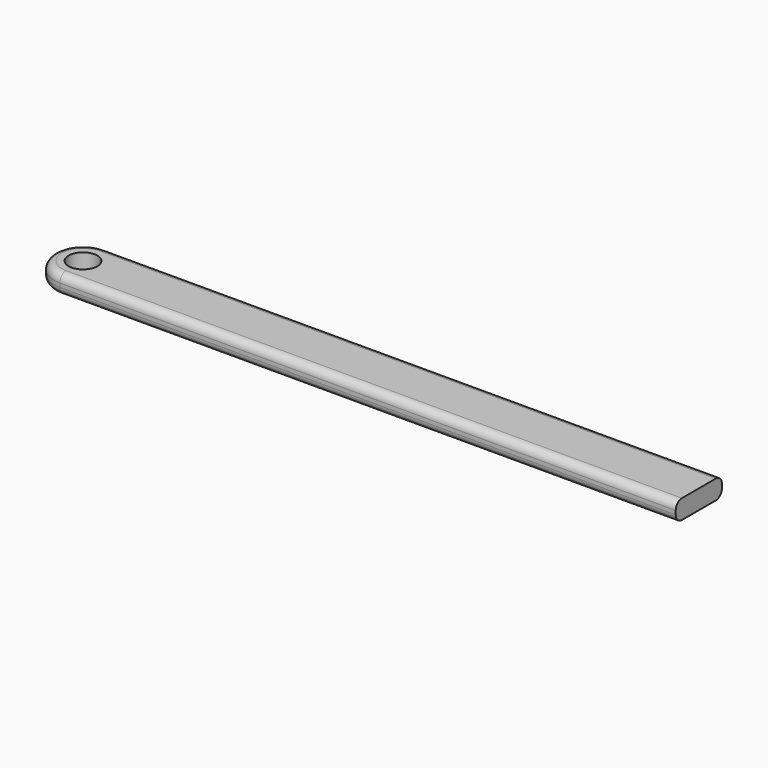
from build123d import *

# Parameters (mm, degrees)
F0_R     = 4.7625
F2_DEPTH = 3.175
F3_R     = 2.54


# Not quite as in the source:
# - a variable given as a bare number and used for a length is read in inches; the dataset says mm whatever the document's units were


with BuildPart() as f2:
    # F0 (on Top) → F2 (new body, symmetric)
    with BuildSketch(Plane.XY):
        with BuildLine():
            Line((-203.2, 0), (0, 0))
            Line((0, 0), (0, 19.05))
            Line((0, 19.05), (-203.2, 19.05))
            ThreePointArc((-203.2, 19.05), (-212.725, 9.525), (-203.2, 0))
        make_face()
        with Locations((-203.2, 9.525)):
            Circle(F0_R, mode=Mode.SUBTRACT)
    extrude(amount=F2_DEPTH, both=True)

    # F3
    f3_edges = [f2.edges().sort_by_distance(p)[0] for p in [
        (-101.6, 0, 3.175),
        (-101.6, 0, -3.175),
    ]]
    fillet(f3_edges, radius=F3_R)


solid = f2.part
